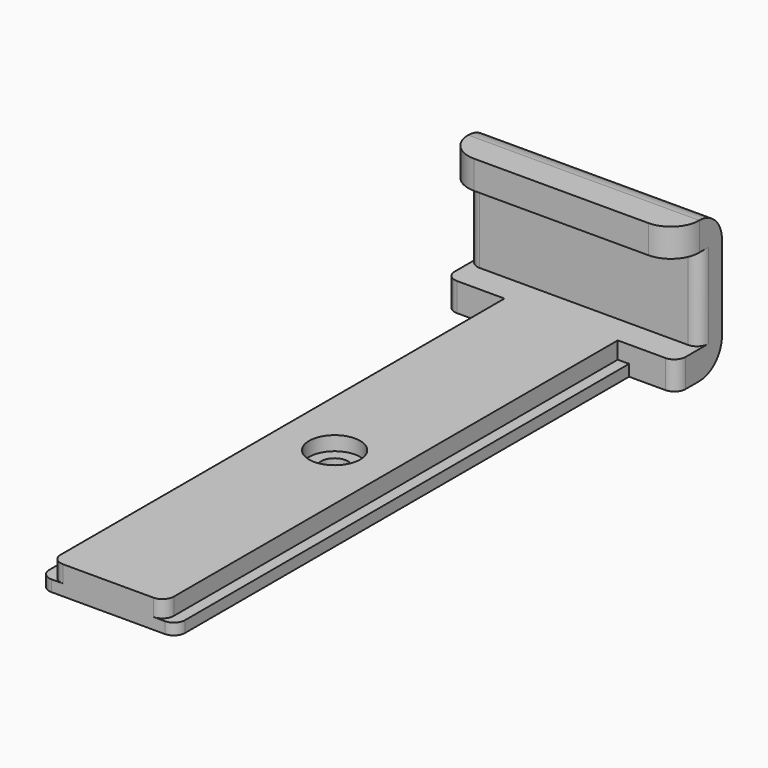
from build123d import *

# Parameters (mm, degrees)
F0_R     = 4.5
F0_R_2   = 2.4
F1_DEPTH = 2.5
F2_DEPTH = 5
F0_W     = 2
F0_H     = 100
F3_DEPTH = 2
F4_W     = 40.8
F4_H     = 5
F5_DEPTH = 15
F6_W     = 40.8
F6_H     = 10
F7_DEPTH = 5
F8_R     = 4.99999
F9_R     = 2


# Not quite as in the source:
# - a fillet or chamfer is up to 0.001 mm smaller than in the source, because OpenCascade refuses the exact size


with BuildPart() as f1:
    # F0 (on Top) → F1 (new body)
    with BuildSketch(Plane.XY):
        Circle(F0_R)
        Circle(F0_R_2, mode=Mode.SUBTRACT)
    extrude(amount=F1_DEPTH)

    # F0 (on Top) → F2 (join)
    with BuildSketch(Plane.XY):
        Polygon((-10, -50), (10, -50), (10, 50), (0, 50), (-10, 50), align=None)
        Circle(F0_R, mode=Mode.SUBTRACT)
        Polygon((0, 50), (10, 50), (12, 50), (20.4, 50), (20.4, 60), (-20.4, 60), (-20.4, 50), (-12, 50), (-10, 50), align=None)
    extrude(amount=F2_DEPTH)

    # F0 (on Top) → F3 (join)
    with BuildSketch(Plane.XY):
        with Locations((-11, 0)):
            Rectangle(F0_W, F0_H)
        with Locations((11, 0)):
            Rectangle(F0_W, F0_H)
    extrude(amount=F3_DEPTH)

    # F4 (on face) → F5 (join)
    with BuildSketch(Plane.XY.offset(5)):
        with Locations((0, 57.5)):
            Rectangle(F4_W, F4_H)
    extrude(amount=F5_DEPTH)

    # F6 (on face) → F7 (join)
    with BuildSketch(Plane.XY.offset(20)):
        with Locations((0, 55)):
            Rectangle(F6_W, F6_H)
    extrude(amount=F7_DEPTH)

    # F8 (radius 5 in the source; OpenCascade refuses exactly that, so slightly less here)
    f8_edges = [f1.edges().sort_by_distance(p)[0] for p in [
        (-20.4, 50, 22.5),
        (20.4, 50, 22.5),
        (0, 60, 25),
        (0, 60, 0),
    ]]
    fillet(f8_edges, radius=F8_R)

    # F9
    f9_edges = [f1.edges().sort_by_distance(p)[0] for p in [
        (-20.4, 55, 12.5),
        (20.4, 55, 12.5),
        (-12, -50, 1),
        (12, -50, 1),
        (-10, -50, 3.5),
        (10, -50, 3.5),
        (-20.4, 50, 2.5),
        (20.4, 50, 2.5),
    ]]
    fillet(f9_edges, radius=F9_R)


solid = f1.part
